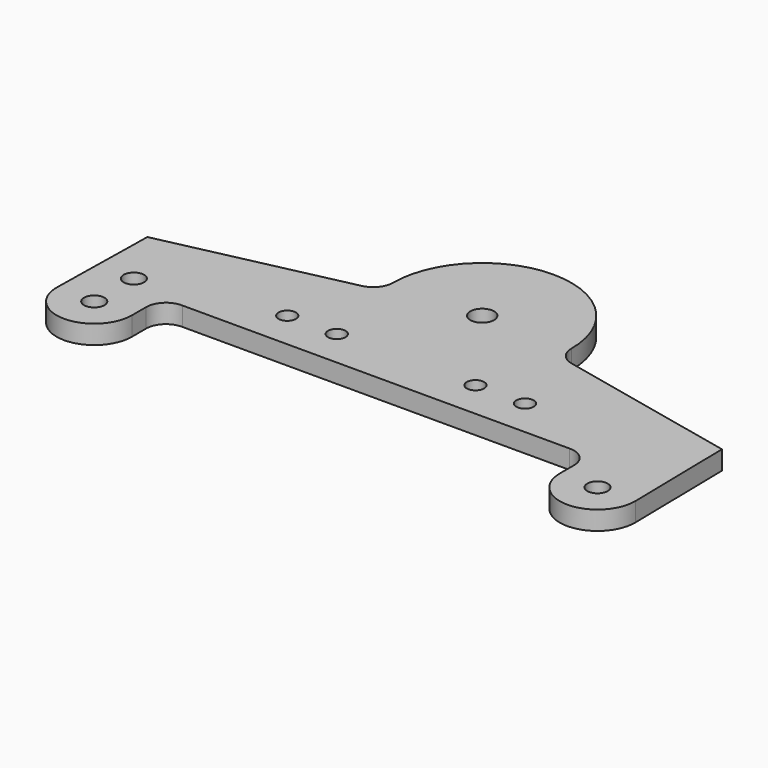
from build123d import *

# Parameters (mm, degrees)
F1_DEPTH = 9.525
F2_D     = 10.3
F3_D     = 8.8
F4_D     = 12
F5_ANGLE = 90


# Not quite as in the source:
# - a length typed as a fraction of an inch, garbled in the dataset ("3 / 203.2 mm" for 3/8 in), is restored
# - a feature names something its author has since deleted; it is built from what else it names


with BuildPart() as f1:
    # F0 (on Front) → F1 (new body)
    with BuildSketch(Plane.XZ):
        with BuildLine():
            ThreePointArc((-108, -36.0045329175), (-104.9318381582, -28.796924455), (-97.6100760503, -26.0121378435))
            Line((-97.6100760503, -26.0121378435), (0, -26.0121378435))
            Line((0, -26.0121378435), (97.6100760503, -26.0121378435))
            ThreePointArc((97.6100760503, -26.0121378435), (104.9318381582, -28.796924455), (108, -36.0045329175))
            Line((108, -36.0045329175), (108, -45.0045329175))
            ThreePointArc((108, -45.0045329175), (127.1790782013, -64.0036889776), (145.9966243156, -44.6463924235))
            Line((145.9966243156, -44.6463924235), (145, 10.9954670825))
            Line((145, 10.9954670825), (52.8553396226, 31.2281526171))
            ThreePointArc((52.8553396226, 31.2281526171), (47.2074842389, 34.7283546603), (45, 40.9954670825))
            ThreePointArc((45, 40.9954670825), (31.8198051534, 72.8152722359), (0, 85.9954670825))
            ThreePointArc((0, 85.9954670825), (-31.8198051534, 72.8152722359), (-45, 40.9954670825))
            ThreePointArc((-45, 40.9954670825), (-47.2074842389, 34.7283546603), (-52.8553396226, 31.2281526171))
            Line((-52.8553396226, 31.2281526171), (-145, 10.9954670825))
            Line((-145, 10.9954670825), (-145.9966243156, -44.6463924235))
            ThreePointArc((-145.9966243156, -44.6463924235), (-127.1790782013, -64.0036889776), (-108, -45.0045329175))
            Line((-108, -45.0045329175), (-108, -36.0045329175))
        make_face()
    extrude(amount=-F1_DEPTH)

    # F2 (through all)
    with Locations(Plane.XZ):
        with Locations((-127, -45.0045329175), (-127, -20.0045329175), (127, -45.0045329175)):
            Hole(F2_D / 2)

    # F3 (through all)
    with Locations(Plane.XZ):
        with Locations((-60, -7.0045329175), (-35, -7.0045329175), (35, -7.0045329175), (60, -7.0045329175)):
            Hole(F3_D / 2)

    # F4 (through all)
    with Locations(Plane.XZ):
        with Locations((0, 40.9954670825)):
            Hole(F4_D / 2)


with BuildPart() as f1_1:
    # F5: moved
    add(f1.part.rotate(Axis((-53.975, 0, -64.0045329175), (-1, 0, 0)), F5_ANGLE))


solid = f1_1.part
